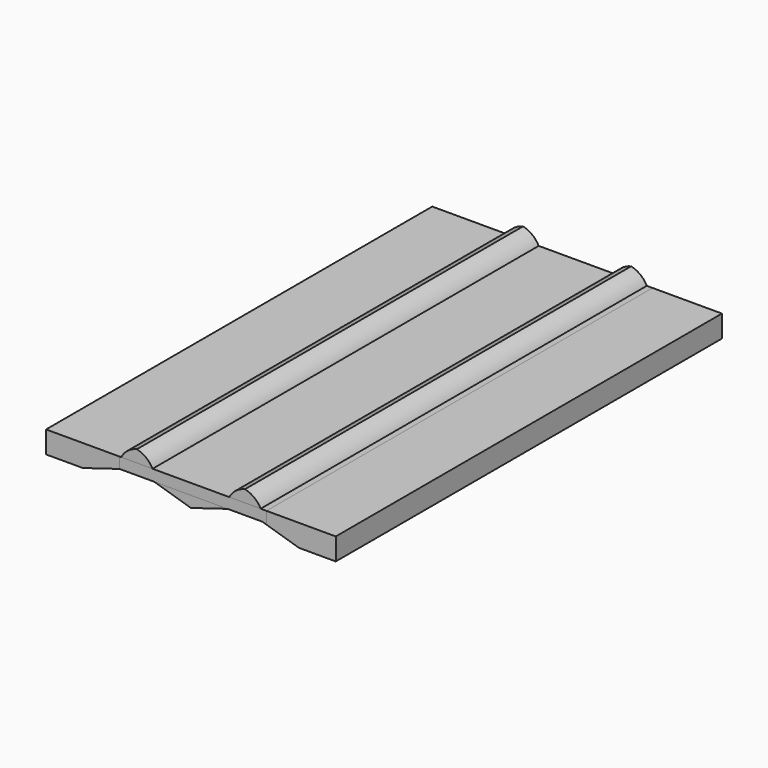
from build123d import *

# Parameters (mm, degrees)
F0_W        = 12.7
F0_H        = 83.4571514838
F1_DEPTH    = 10.16
F0_W_2      = 6.35
F2_DEPTH    = 11.43
F3_T1_DEPTH = 103.7771514838
F4_T1_DEPTH = 103.7771514838
F5_DEPTH    = 6.35
F8_DEPTH    = 54.356
F18_DEPTH   = 25.4


# Not quite as in the source:
# - a fillet or chamfer that OpenCascade refuses, or shapes differently, is made with other operations: its cross-section is extruded or revolved along the edge and cut away or added


with BuildPart() as f1:
    # F0 (on Top) → F1 (new body)
    with BuildSketch(Plane.XY):
        with Locations((16.1417351018, -1.7268359661)):
            Rectangle(F0_W, F0_H)
    extrude(amount=F1_DEPTH)


with BuildPart() as f1b:
    # F0 (on Top) → F1, piece 2 (new body)
    with BuildSketch(Plane.XY):
        with Locations((-2.9082648982, -1.7268359661)):
            Rectangle(F0_W, F0_H)
    extrude(amount=F1_DEPTH)


with BuildPart() as f1c:
    # F0 (on Top) → F1, piece 3 (new body)
    with BuildSketch(Plane.XY):
        with Locations((-21.9582648982, -1.7268359661)):
            Rectangle(F0_W, F0_H)
    extrude(amount=F1_DEPTH)


with BuildPart() as f2:
    # F0 (on Top) → F2 (new body)
    with BuildSketch(Plane.XY):
        with Locations((-12.4332648982, -1.7268359661)):
            Rectangle(F0_W_2, F0_H)
    extrude(amount=F2_DEPTH)

    # F4: fillet of radius 4.064 on 2 edges, made by hand

    # F4_s2 → F4_t1 (cut)
    with BuildSketch(Plane.XZ.offset(-50.1617397758)):
        with BuildLine():
            ThreePointArc((-9.2582648982, 7.366), (-10.4485829395, 10.2396819587), (-13.3222648982, 11.43))
            Line((-13.3222648982, 11.43), (-9.2582648982, 11.43))
            Line((-9.2582648982, 11.43), (-9.2582648982, 7.366))
        make_face()
        with BuildLine():
            ThreePointArc((-15.6082648982, 7.366), (-14.417946857, 10.2396819587), (-11.5442648982, 11.43))
            Line((-11.5442648982, 11.43), (-15.6082648982, 11.43))
            Line((-15.6082648982, 11.43), (-15.6082648982, 7.366))
        make_face()
    extrude(amount=F4_T1_DEPTH, mode=Mode.SUBTRACT)


with BuildPart() as f2b:
    # F0 (on Top) → F2, piece 2 (new body)
    with BuildSketch(Plane.XY):
        with Locations((6.6167351018, -1.7268359661)):
            Rectangle(F0_W_2, F0_H)
    extrude(amount=F2_DEPTH)

    # F3: fillet of radius 4.064 on 2 edges, made by hand

    # F3_s2 → F3_t1 (cut)
    with BuildSketch(Plane.XZ.offset(-50.1617397758)):
        with BuildLine():
            ThreePointArc((9.7917351018, 7.366), (8.6014170605, 10.2396819587), (5.7277351018, 11.43))
            Line((5.7277351018, 11.43), (9.7917351018, 11.43))
            Line((9.7917351018, 11.43), (9.7917351018, 7.366))
        make_face()
        with BuildLine():
            ThreePointArc((3.4417351018, 7.366), (4.632053143, 10.2396819587), (7.5057351018, 11.43))
            Line((7.5057351018, 11.43), (3.4417351018, 11.43))
            Line((3.4417351018, 11.43), (3.4417351018, 7.366))
        make_face()
    extrude(amount=F3_T1_DEPTH, mode=Mode.SUBTRACT)


with BuildPart() as f5:
    # F0 (on Top) → F5 (new body)
    with BuildSketch(Plane.XY):
        with Locations((-21.9582648982, -1.7268359661)):
            Rectangle(F0_W, F0_H)
        with Locations((-12.4332648982, -1.7268359661)):
            Rectangle(F0_W_2, F0_H)
        with Locations((-2.9082648982, -1.7268359661)):
            Rectangle(F0_W, F0_H)
        with Locations((6.6167351018, -1.7268359661)):
            Rectangle(F0_W_2, F0_H)
        with Locations((16.1417351018, -1.7268359661)):
            Rectangle(F0_W, F0_H)
    extrude(amount=F5_DEPTH)


with BuildPart() as f1_1:
    add(f1.part)

    # F6: cut F5
    add(f5.part, mode=Mode.SUBTRACT)


with BuildPart() as f2b_1:
    add(f2b.part)

    # F6: cut F5
    add(f5.part, mode=Mode.SUBTRACT)


with BuildPart() as f1b_1:
    add(f1b.part)

    # F6: cut F5
    add(f5.part, mode=Mode.SUBTRACT)


with BuildPart() as f2_1:
    add(f2.part)

    # F6: cut F5
    add(f5.part, mode=Mode.SUBTRACT)


with BuildPart() as f1c_1:
    add(f1c.part)

    # F6: cut F5
    add(f5.part, mode=Mode.SUBTRACT)


with BuildPart() as f8:
    # F7 (on Front) → F8 (new body, symmetric)
    with BuildSketch(Plane.XZ):
        Polygon((5.4737351018, 8.89), (-2.9082648982, 6.35), (16.1417351018, 6.35), (7.7597351018, 8.89), align=None)
    extrude(amount=F8_DEPTH, both=True)


with BuildPart() as f8b:
    # F7 (on Front) → F8, piece 2 (new body, symmetric)
    with BuildSketch(Plane.XZ):
        Polygon((-2.9082648982, 6.35), (-11.2902648982, 8.89), (-13.5762648982, 8.89), (-21.9582648982, 6.35), align=None)
    extrude(amount=F8_DEPTH, both=True)


with BuildPart() as f1_2:
    add(f1_1.part)

    # F9: cut F8, F8b
    add(f8.part, mode=Mode.SUBTRACT)
    add(f8b.part, mode=Mode.SUBTRACT)


with BuildPart() as f2b_2:
    add(f2b_1.part)

    # F9: cut F8, F8b
    add(f8.part, mode=Mode.SUBTRACT)
    add(f8b.part, mode=Mode.SUBTRACT)


with BuildPart() as f1b_2:
    add(f1b_1.part)

    # F9: cut F8, F8b
    add(f8.part, mode=Mode.SUBTRACT)
    add(f8b.part, mode=Mode.SUBTRACT)


with BuildPart() as f2_2:
    add(f2_1.part)

    # F9: cut F8, F8b
    add(f8.part, mode=Mode.SUBTRACT)
    add(f8b.part, mode=Mode.SUBTRACT)


with BuildPart() as f1c_2:
    add(f1c_1.part)

    # F9: cut F8, F8b
    add(f8.part, mode=Mode.SUBTRACT)
    add(f8b.part, mode=Mode.SUBTRACT)


with BuildPart() as f1_3:
    # F10: moved
    add(f1_2.part.moved(Location((2.54, 0, 0))))


with BuildPart() as f1c_3:
    # F10: moved
    add(f1c_2.part.moved(Location((2.54, 0, 0))))


with BuildPart() as f1b_3:
    # F10: moved
    add(f1b_2.part.moved(Location((2.54, 0, 0))))


with BuildPart() as f2_3:
    # F10: moved
    add(f2_2.part.moved(Location((2.54, 0, 0))))


with BuildPart() as f2b_3:
    # F10: moved
    add(f2b_2.part.moved(Location((2.54, 0, 0))))


with BuildPart() as f1_4:
    # F11: moved
    add(f1_3.part.moved(Location((0.254, 0, 0))))


with BuildPart() as f1c_4:
    # F11: moved
    add(f1c_3.part.moved(Location((0.254, 0, 0))))


with BuildPart() as f1b_4:
    # F11: moved
    add(f1b_3.part.moved(Location((0.254, 0, 0))))


with BuildPart() as f2_4:
    # F11: moved
    add(f2_3.part.moved(Location((0.254, 0, 0))))


with BuildPart() as f2b_4:
    # F11: moved
    add(f2b_3.part.moved(Location((0.254, 0, 0))))


with BuildPart() as f2_5:
    # F12: moved
    add(f2_4.part.moved(Location((0, 0, 0.9144))))


with BuildPart() as f1c_5:
    # F13: moved
    add(f1c_4.part.moved(Location((0.1778, 0, 0))))


with BuildPart() as f1c_6:
    # F14: moved
    add(f1c_5.part.moved(Location((0.1778, 0, 0))))


with BuildPart() as f2_6:
    # F14: moved
    add(f2_5.part.moved(Location((0.1778, 0, 0))))


with BuildPart() as f2b_5:
    # F15: moved
    add(f2b_4.part.moved(Location((0, 0, 0.9144))))


with BuildPart() as f1b_5:
    # F16: moved
    add(f1b_4.part.moved(Location((0.1778, 0, 0))))


with BuildPart() as f2_7:
    # F16: moved
    add(f2_6.part.moved(Location((0.1778, 0, 0))))


with BuildPart() as f1c_7:
    # F16: moved
    add(f1c_6.part.moved(Location((0.1778, 0, 0))))


with BuildPart() as f1c_8:
    # F17: moved
    add(f1c_7.part.moved(Location((0.1778, 0, 0))))


with BuildPart() as f2_8:
    # F17: moved
    add(f2_7.part.moved(Location((0.1778, 0, 0))))


with BuildPart() as f1b_6:
    # F17: moved
    add(f1b_5.part.moved(Location((0.1778, 0, 0))))


with BuildPart() as f2b_6:
    # F17: moved
    add(f2b_5.part.moved(Location((0.1778, 0, 0))))


with BuildPart() as f18:
    # F18 (new): a face of the model
    f18_faces = [f1c_8.part.faces().sort_by_distance(p)[0] for p in [
        (-12.1030648982, -1.7268359661, 9.2171212121),
    ]]
    extrude(f18_faces, amount=F18_DEPTH)


solid = Compound([f1_4.part, f1c_8.part, f2_8.part, f1b_6.part, f2b_6.part, f18.part])
